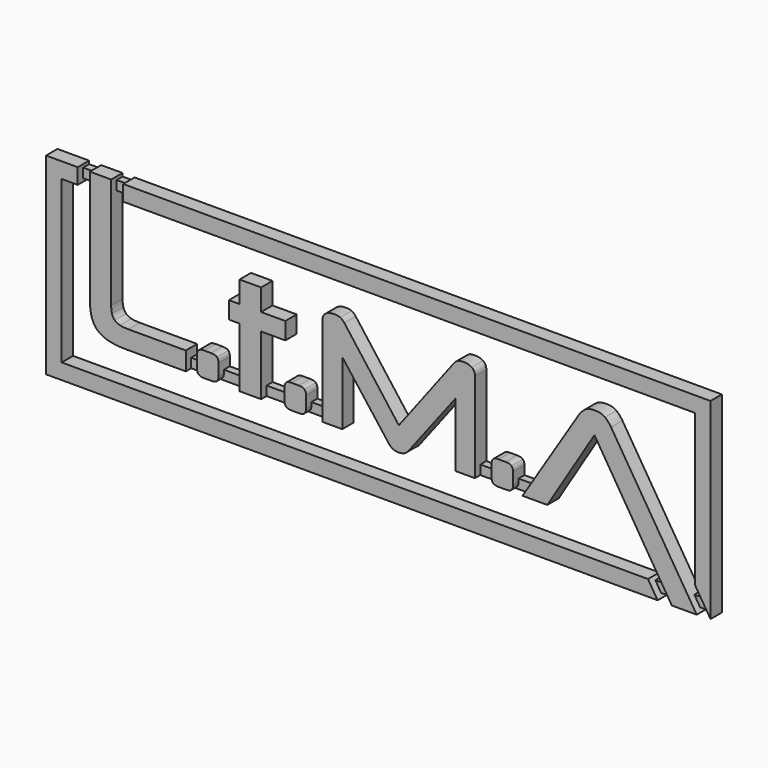
from build123d import *

# Parameters (mm, degrees)
F1_DEPTH = 3.81
F2_W     = 12.1664756684
F2_H     = 2.5
F3_DEPTH = 2


# Not quite as in the source:
# - ends of sketch curves that miss each other by under 0.0002 mm in the source are joined


with BuildPart() as f1:
    # F0 (on Front) → F1 (new body)
    with BuildSketch(Plane.XZ):
        with BuildLine():
            Line((-208.6418906424, -101.2208287439), (-214.3634929308, -101.2208287439))
            Line((-214.3634929308, -101.2208287439), (-214.3634929308, -131.0546462962))
            add(Edge.make_bspline(
                [(-214.3634929308, -131.0546462962), (-214.3634929308, -132.6966873023), (-214.2061473092, -134.0798212834), (-213.8903111369, -135.2034824316)],
                knots=[0, 0, 0, 0, 1, 1, 1, 1], degree=3))
            add(Edge.make_bspline(
                [(-213.8903111369, -135.2034824316), (-213.5738803117, -136.3277249196), (-213.0372969724, -137.2376771068), (-212.2793873449, -137.9316082867)],
                knots=[0, 0, 0, 0, 1, 1, 1, 1], degree=3))
            add(Edge.make_bspline(
                [(-212.2793873449, -137.9316082867), (-211.5214777174, -138.627285705), (-210.5117148029, -139.131569181), (-209.2483346124, -139.447423104)],
                knots=[0, 0, 0, 0, 1, 1, 1, 1], degree=3))
            add(Edge.make_bspline(
                [(-209.2483346124, -139.447423104), (-207.9849544218, -139.7632614951), (-206.4063193989, -139.9211884566), (-204.5118393284, -139.9211884566)],
                knots=[0, 0, 0, 0, 1, 1, 1, 1], degree=3))
            Line((-204.5118393284, -139.9211884566), (-188.6726404251, -139.9211884566))
            Line((-188.6726404251, -139.9211884566), (-188.6726404251, -134.9956467782))
            Line((-188.6726404251, -134.9956467782), (-204.0192869356, -134.9956467782))
            add(Edge.make_bspline(
                [(-204.0192869356, -134.9956467782), (-204.9286600018, -134.9956467782), (-205.680112763, -134.9192627156), (-206.2736407815, -134.7678769369)],
                knots=[0, 0, 0, 0, 1, 1, 1, 1], degree=3))
            add(Edge.make_bspline(
                [(-206.2736407815, -134.7678769369), (-206.8677567965, -134.6164401244), (-207.3409385904, -134.3698299905), (-207.6943554995, -134.0293312517)],
                knots=[0, 0, 0, 0, 1, 1, 1, 1], degree=3))
            add(Edge.make_bspline(
                [(-207.6943554995, -134.0293312517), (-208.0483581862, -133.6876498634), (-208.2949305996, -133.2591003257), (-208.4334803057, -132.7407027169)],
                knots=[0, 0, 0, 0, 1, 1, 1, 1], degree=3))
            add(Edge.make_bspline(
                [(-208.4334803057, -132.7407027169), (-208.5726180082, -132.2235055084), (-208.6418906424, -131.5847572373), (-208.6418906424, -130.8268587041)],
                knots=[0, 0, 0, 0, 1, 1, 1, 1], degree=3))
            Line((-208.6418906424, -130.8268587041), (-208.6418906424, -101.2208287439))
        make_face()
    extrude(amount=F1_DEPTH)



with BuildPart() as f1b:
    # F0 (on Front) → F1, piece 2 (new body)
    with BuildSketch(Plane.XZ):
        with BuildLine():
            add(Edge.make_bspline(
                [(-185.2435518405, -133.8203306997), (-185.5347409782, -134.0986083236), (-185.6797475505, -134.527756952), (-185.6797475505, -135.1089592344)],
                knots=[0, 0, 0, 0, 1, 1, 1, 1], degree=3))
            Line((-185.6797475505, -135.1089592344), (-185.6797475505, -138.2157436862))
            add(Edge.make_bspline(
                [(-185.6797475505, -138.2157436862), (-185.6797475505, -138.8227712149), (-185.5347343216, -139.2577953698), (-185.2435518405, -139.5231592611)],
                knots=[0, 0, 0, 0, 1, 1, 1, 1], degree=3))
            add(Edge.make_bspline(
                [(-185.2435518405, -139.5231592611), (-184.9535409146, -139.7885054015), (-184.4551152143, -139.9211884566), (-183.7471054033, -139.9211884566)],
                knots=[0, 0, 0, 0, 1, 1, 1, 1], degree=3))
            Line((-183.7471054033, -139.9211884566), (-181.8901971941, -139.9211884566))
            add(Edge.make_bspline(
                [(-181.8901971941, -139.9211884566), (-181.1581194695, -139.9211884566), (-180.6467800366, -139.7885564352), (-180.355590899, -139.5231592611)],
                knots=[0, 0, 0, 0, 1, 1, 1, 1], degree=3))
            add(Edge.make_bspline(
                [(-180.355590899, -139.5231592611), (-180.0655777542, -139.2577953698), (-179.9199854042, -138.8227712149), (-179.9199854042, -138.2157436862)],
                knots=[0, 0, 0, 0, 1, 1, 1, 1], degree=3))
            Line((-179.9199854042, -138.2157436862), (-179.9199854042, -135.1089592344))
            add(Edge.make_bspline(
                [(-179.9199854042, -135.1089592344), (-179.9199854042, -134.527756952), (-180.0655799731, -134.0986083236), (-180.355590899, -133.8203306997)],
                knots=[0, 0, 0, 0, 1, 1, 1, 1], degree=3))
            add(Edge.make_bspline(
                [(-180.355590899, -133.8203306997), (-180.6467800366, -133.5432357252), (-181.1581194695, -133.403514464), (-181.8901971941, -133.403514464)],
                knots=[0, 0, 0, 0, 1, 1, 1, 1], degree=3))
            Line((-181.8901971941, -133.403514464), (-183.7471054033, -133.403514464))
            add(Edge.make_bspline(
                [(-183.7471054033, -133.403514464), (-184.4551152143, -133.403514464), (-184.9535409146, -133.5433022908), (-185.2435518405, -133.8203306997)],
                knots=[0, 0, 0, 0, 1, 1, 1, 1], degree=3))
        make_face()
    extrude(amount=F1_DEPTH)


with BuildPart() as f1c:
    # F0 (on Front) → F1, piece 3 (new body)
    with BuildSketch(Plane.XZ):
        Polygon((-168.5149384664, -113.5863090252), (-174.2747006127, -113.5863090252), (-174.2747006127, -119.3842421237), (-177.1542899065, -119.3842421237), (-177.1542899065, -123.9686837538), (-174.2747006127, -123.9686837538), (-174.2747006127, -139.9211884566), (-168.5149384664, -139.9211884566), (-168.5149384664, -123.9686837538), (-162.0360145469, -123.9686837538), (-162.0360145469, -119.3842421237), (-168.5149384664, -119.3842421237), align=None)
    extrude(amount=F1_DEPTH)


with BuildPart() as f1d:
    # F0 (on Front) → F1, piece 4 (new body)
    with BuildSketch(Plane.XZ):
        with BuildLine():
            add(Edge.make_bspline(
                [(-161.8264282174, -133.8203306997), (-162.117617355, -134.0986083236), (-162.2626239274, -134.527756952), (-162.2626239274, -135.1089592344)],
                knots=[0, 0, 0, 0, 1, 1, 1, 1], degree=3))
            Line((-162.2626239274, -135.1089592344), (-162.2626239274, -138.2157436862))
            add(Edge.make_bspline(
                [(-162.2626239274, -138.2157436862), (-162.2626239274, -138.8227712149), (-162.1176106984, -139.2577953698), (-161.8264282174, -139.5231592611)],
                knots=[0, 0, 0, 0, 1, 1, 1, 1], degree=3))
            add(Edge.make_bspline(
                [(-161.8264282174, -139.5231592611), (-161.5364150726, -139.7885054015), (-161.0379915911, -139.9211884566), (-160.3299839989, -139.9211884566)],
                knots=[0, 0, 0, 0, 1, 1, 1, 1], degree=3))
            Line((-160.3299839989, -139.9211884566), (-158.4730757898, -139.9211884566))
            add(Edge.make_bspline(
                [(-158.4730757898, -139.9211884566), (-157.7409958463, -139.9211884566), (-157.2296564134, -139.7885564352), (-156.9384694947, -139.5231592611)],
                knots=[0, 0, 0, 0, 1, 1, 1, 1], degree=3))
            add(Edge.make_bspline(
                [(-156.9384694947, -139.5231592611), (-156.648454131, -139.2577953698), (-156.5028617811, -138.8227712149), (-156.5028617811, -138.2157436862)],
                knots=[0, 0, 0, 0, 1, 1, 1, 1], degree=3))
            Line((-156.5028617811, -138.2157436862), (-156.5028617811, -135.1089592344))
            add(Edge.make_bspline(
                [(-156.5028617811, -135.1089592344), (-156.5028617811, -134.527756952), (-156.6484563499, -134.0986083236), (-156.9384694947, -133.8203306997)],
                knots=[0, 0, 0, 0, 1, 1, 1, 1], degree=3))
            add(Edge.make_bspline(
                [(-156.9384694947, -133.8203306997), (-157.2296564134, -133.5432357252), (-157.7409958463, -133.403514464), (-158.4730757898, -133.403514464)],
                knots=[0, 0, 0, 0, 1, 1, 1, 1], degree=3))
            Line((-158.4730757898, -133.403514464), (-160.3299839989, -133.403514464))
            add(Edge.make_bspline(
                [(-160.3299839989, -133.403514464), (-161.0379915911, -133.403514464), (-161.5364150726, -133.5433022908), (-161.8264282174, -133.8203306997)],
                knots=[0, 0, 0, 0, 1, 1, 1, 1], degree=3))
        make_face()
    extrude(amount=F1_DEPTH)


with BuildPart() as f1e:
    # F0 (on Front) → F1, piece 5 (new body)
    with BuildSketch(Plane.XZ):
        with BuildLine():
            add(Edge.make_bspline(
                [(-115.9362036674, -113.7947260185), (-116.3019485316, -113.9843559716), (-116.6494854765, -114.2937352775), (-116.9770727016, -114.7234674647)],
                knots=[0, 0, 0, 0, 1, 1, 1, 1], degree=3))
            Line((-116.9770727016, -114.7234674647), (-131.6656114364, -134.085694591))
            Line((-131.6656114364, -134.085694591), (-146.2396750352, -114.7234674647))
            add(Edge.make_bspline(
                [(-146.2396750352, -114.7234674647), (-146.5678413813, -114.2937352775), (-146.9341786795, -113.9843559716), (-147.3380834015, -113.7947260185)],
                knots=[0, 0, 0, 0, 1, 1, 1, 1], degree=3))
            add(Edge.make_bspline(
                [(-147.3380834015, -113.7947260185), (-147.7414001271, -113.6050982842), (-148.2844425516, -113.5099915283), (-148.9654466858, -113.5099915283)],
                knots=[0, 0, 0, 0, 1, 1, 1, 1], degree=3))
            add(Edge.make_bspline(
                [(-148.9654466858, -113.5099915283), (-149.8489878491, -113.5099915283), (-150.5875268778, -113.6996214814), (-151.1810548963, -114.0794605087)],
                knots=[0, 0, 0, 0, 1, 1, 1, 1], degree=3))
            add(Edge.make_bspline(
                [(-151.1810548963, -114.0794605087), (-151.7739993562, -114.4581191054), (-152.0704693672, -115.0516515616), (-152.0704693672, -115.8600423454)],
                knots=[0, 0, 0, 0, 1, 1, 1, 1], degree=3))
            Line((-152.0704693672, -115.8600423454), (-152.0704693672, -139.9211884566))
            Line((-152.0704693672, -139.9211884566), (-146.8032684891, -139.9211884566))
            Line((-146.8032684891, -139.9211884566), (-146.8032684891, -122.90784503))
            Line((-146.8032684891, -122.90784503), (-134.2393383084, -139.390476206))
            add(Edge.make_bspline(
                [(-134.2393383084, -139.390476206), (-133.6587195848, -140.1225494929), (-132.8133360605, -140.4894747876), (-131.7037712942, -140.4894747876)],
                knots=[0, 0, 0, 0, 1, 1, 1, 1], degree=3))
            add(Edge.make_bspline(
                [(-131.7037712942, -140.4894747876), (-130.5930394106, -140.4894747876), (-129.7482372262, -140.1225494929), (-129.1676185025, -139.390476206)],
                knots=[0, 0, 0, 0, 1, 1, 1, 1], degree=3))
            Line((-129.1676185025, -139.390476206), (-116.5655306828, -122.90784503))
            Line((-116.5655306828, -122.90784503), (-116.5655306828, -139.9211884566))
            Line((-116.5655306828, -139.9211884566), (-111.298325367, -139.9211884566))
            Line((-111.298325367, -139.9211884566), (-111.298325367, -115.8600423454))
            add(Edge.make_bspline(
                [(-111.298325367, -115.8600423454), (-111.298325367, -115.0516515616), (-111.595390031, -114.4581191054), (-112.1883233966, -114.0794605087)],
                knots=[0, 0, 0, 0, 1, 1, 1, 1], degree=3))
            add(Edge.make_bspline(
                [(-112.1883233966, -114.0794605087), (-112.7818558528, -113.6996214814), (-113.5192211075, -113.5099915283), (-114.4027622708, -113.5099915283)],
                knots=[0, 0, 0, 0, 1, 1, 1, 1], degree=3))
            add(Edge.make_bspline(
                [(-114.4027622708, -113.5099915283), (-115.0597007103, -113.5099915283), (-115.5704565845, -113.6051803818), (-115.9362036674, -113.7947260185)],
                knots=[0, 0, 0, 0, 1, 1, 1, 1], degree=3))
        make_face()
    extrude(amount=F1_DEPTH)


with BuildPart() as f1f:
    # F0 (on Front) → F1, piece 6 (new body)
    with BuildSketch(Plane.XZ):
        with BuildLine():
            add(Edge.make_bspline(
                [(-106.4303318961, -133.8203306997), (-106.7209241619, -134.0986083236), (-106.8653538321, -134.527756952), (-106.8653538321, -135.1089592344)],
                knots=[0, 0, 0, 0, 1, 1, 1, 1], degree=3))
            Line((-106.8653538321, -135.1089592344), (-106.8653538321, -138.2157436862))
            add(Edge.make_bspline(
                [(-106.8653538321, -138.2157436862), (-106.8653538321, -138.8227712149), (-106.720906411, -139.2577953698), (-106.4303318961, -139.5231592611)],
                knots=[0, 0, 0, 0, 1, 1, 1, 1], degree=3))
            add(Edge.make_bspline(
                [(-106.4303318961, -139.5231592611), (-106.1403209702, -139.7885054015), (-105.6407126204, -139.9211884566), (-104.9332863681, -139.9211884566)],
                knots=[0, 0, 0, 0, 1, 1, 1, 1], degree=3))
            Line((-104.9332863681, -139.9211884566), (-103.0769705931, -139.9211884566))
            add(Edge.make_bspline(
                [(-103.0769705931, -139.9211884566), (-102.3443004344, -139.9211884566), (-101.8329765334, -139.7885564352), (-101.5417829581, -139.5231592611)],
                knots=[0, 0, 0, 0, 1, 1, 1, 1], degree=3))
            add(Edge.make_bspline(
                [(-101.5417829581, -139.5231592611), (-101.2523578097, -139.2577953698), (-101.1061774634, -138.8227712149), (-101.1061774634, -138.2157436862)],
                knots=[0, 0, 0, 0, 1, 1, 1, 1], degree=3))
            Line((-101.1061774634, -138.2157436862), (-101.1061774634, -135.1089592344))
            add(Edge.make_bspline(
                [(-101.1061774634, -135.1089592344), (-101.1061774634, -134.527756952), (-101.2522890252, -134.0986083236), (-101.5417829581, -133.8203306997)],
                knots=[0, 0, 0, 0, 1, 1, 1, 1], degree=3))
            add(Edge.make_bspline(
                [(-101.5417829581, -133.8203306997), (-101.8329765334, -133.5432357252), (-102.3443004344, -133.403514464), (-103.0769705931, -133.403514464)],
                knots=[0, 0, 0, 0, 1, 1, 1, 1], degree=3))
            Line((-103.0769705931, -133.403514464), (-104.9332863681, -133.403514464))
            add(Edge.make_bspline(
                [(-104.9332863681, -133.403514464), (-105.6407126204, -133.403514464), (-106.1403209702, -133.5433022908), (-106.4303318961, -133.8203306997)],
                knots=[0, 0, 0, 0, 1, 1, 1, 1], degree=3))
        make_face()
    extrude(amount=F1_DEPTH)


with BuildPart() as f1g:
    # F0 (on Front) → F1, piece 7 (new body)
    with BuildSketch(Plane.XZ):
        with BuildLine():
            add(Edge.make_bspline(
                [(-81.9335780713, -114.2303315132), (-82.5652703855, -114.7105537321), (-83.10831281, -115.3169999209), (-83.5632889036, -116.0496700797)],
                knots=[0, 0, 0, 0, 1, 1, 1, 1], degree=3))
            Line((-83.5632889036, -116.0496700797), (-98.5682629012, -139.9211884566))
            Line((-98.5682629012, -139.9211884566), (-91.9372786712, -139.9211884566))
            Line((-91.9372786712, -139.9211884566), (-79.3193460123, -119.3460844846))
            Line((-79.3193460123, -119.3460844846), (-58.6191985009, -152.7792388815))
            Line((-58.6191985009, -152.7792388815), (-51.950054413, -152.7792388815))
            Line((-51.950054413, -152.7792388815), (-74.8857753867, -116.0496700797))
            add(Edge.make_bspline(
                [(-74.8857753867, -116.0496700797), (-75.3401701405, -115.3169999209), (-75.8837939048, -114.7105537321), (-76.515486219, -114.2303315132)],
                knots=[0, 0, 0, 0, 1, 1, 1, 1], degree=3))
            add(Edge.make_bspline(
                [(-76.515486219, -114.2303315132), (-77.1465949744, -113.7512764117), (-78.043633429, -113.5099915283), (-79.2054522162, -113.5099915283)],
                knots=[0, 0, 0, 0, 1, 1, 1, 1], degree=3))
            add(Edge.make_bspline(
                [(-79.2054522162, -113.5099915283), (-80.3931006874, -113.5099915283), (-81.3024693159, -113.7512764117), (-81.9335780713, -114.2303315132)],
                knots=[0, 0, 0, 0, 1, 1, 1, 1], degree=3))
        make_face()
    extrude(amount=F1_DEPTH)


with BuildPart() as f1h:
    # F0 (on Front) → F1, piece 8 (new body)
    with BuildSketch(Plane.XZ):
        Polygon((-48.2597245686, -101.2208287439), (-205.419452843, -101.2208287439), (-205.419452843, -105.3907994674), (-52.4302766319, -105.3907994674), (-52.4302766319, -145.926340367), (-48.2597245686, -152.6042866502), align=None)
    extrude(amount=F1_DEPTH)


with BuildPart() as f1i:
    # F0 (on Front) → F1, piece 9 (new body)
    with BuildSketch(Plane.XZ):
        Polygon((-217.5859285114, -101.2208287439), (-226.0597245686, -101.2208287439), (-226.0597245686, -152.7792388815), (-62.4087466384, -152.7792388815), (-64.9912779247, -148.6086690674), (-221.8897538451, -148.6086690674), (-221.8897538451, -105.3907994674), (-217.5859285114, -105.3907994674), align=None)
    extrude(amount=F1_DEPTH)


with BuildPart() as f1_1:
    add(f1.part)

    add(f1b.part)  # F3 merges F1b

    add(f1c.part)  # F3 merges F1c

    add(f1d.part)  # F3 merges F1d

    add(f1e.part)  # F3 merges F1e

    add(f1f.part)  # F3 merges F1f

    add(f1g.part)  # F3 merges F1g

    add(f1h.part)  # F3 merges F1h

    add(f1i.part)  # F3 merges F1i
    # F2 (on face) → F3 (join)
    with BuildSketch(Plane.XZ):
        with Locations((-211.5026906772, -103.3058141056)):
            Rectangle(F2_W, F2_H)
        Polygon((-50.2334349583, -149.4439539745), (-64.4740465867, -149.4439539745), (-62.9259779765, -151.9439539745), (-48.6721195904, -151.9439539745), align=None)
        Polygon((-188.6726404251, -139.9211884566), (-183.7471054033, -139.9211884566), (-185.6797475505, -137.4211884566), (-188.6726404251, -137.4211884566), align=None)
        Polygon((-174.2747006127, -139.9211884566), (-174.2747006127, -137.4211884566), (-179.9199854042, -137.4211884566), (-181.8901971941, -139.9211884566), align=None)
        Polygon((-162.2626239274, -137.4211884566), (-168.5149384664, -137.4211884566), (-168.5149384664, -139.9211884566), (-160.3299839989, -139.9211884566), align=None)
        Polygon((-152.0704693672, -139.9211884566), (-152.0704693672, -137.4211884566), (-156.5028617811, -137.4211884566), (-158.4730757898, -139.9211884566), align=None)
        Polygon((-106.8653538321, -137.4211884566), (-111.298325367, -137.4211884566), (-111.298325367, -139.9211884566), (-104.0051284806, -139.9211884566), align=None)
        Polygon((-101.1061774634, -137.4211884566), (-103.0769705931, -139.9211884566), (-98.5682629012, -139.9211884566), (-96.9968322783, -137.4211884566), align=None)
    extrude(amount=F3_DEPTH)


solid = f1_1.part
